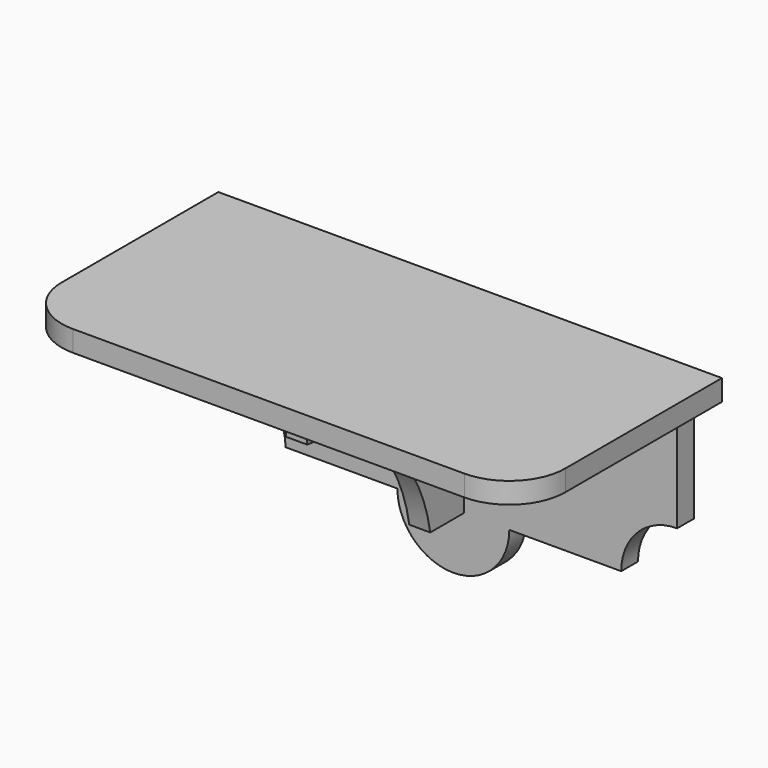
from build123d import *

# Parameters (mm, degrees)
F1_DEPTH = 9.525
F3_DEPTH = 88.9
F5_DEPTH = 9.525
F7_DEPTH = 9.525


# Not quite as in the source:
# - a length typed as a fraction of an inch, garbled in the dataset ("3 / 203.2 mm" for 3/8 in), is restored


with BuildPart() as f1:
    # F0 (on Front) → F1 (new body)
    with BuildSketch(Plane.XZ):
        with BuildLine():
            Line((203.2, 0), (0, 0))
            Line((0, 0), (0, -50.8))
            ThreePointArc((0, -50.8), (17.9605122421, -58.2394877579), (25.4, -76.2))
            Line((25.4, -76.2), (76.2, -76.2))
            ThreePointArc((76.2, -76.2), (101.6, -101.6), (127, -76.2))
            Line((127, -76.2), (177.8, -76.2))
            ThreePointArc((177.8, -76.2), (185.2394877579, -58.2394877579), (203.2, -50.8))
            Line((203.2, -50.8), (203.2, 0))
        make_face()
    extrude(amount=F1_DEPTH)

    # F2 (on face) → F3 (join)
    with BuildSketch(Plane.XZ.offset(9.525)):
        Polygon((96.8375, 0), (96.8375, -76.2), (101.6, -76.2), (106.3625, -76.2), (106.3625, 0), align=None)
    extrude(amount=F3_DEPTH)

    # F4 (on face) → F5 (cut)
    with BuildSketch(Plane.YZ.offset(106.3625)):
        with BuildLine():
            Line((-98.425, -76.2), (-28.575, -76.2))
            ThreePointArc((-28.575, -76.2), (-52.4826849385, -32.3309534324), (-98.425, -12.7))
            Line((-98.425, -12.7), (-98.425, -76.2))
        make_face()
    extrude(amount=-F5_DEPTH, mode=Mode.SUBTRACT)

    # F6 (on face) → F7 (join)
    with BuildSketch(Plane.XY):
        with BuildLine():
            Line((0, -9.525), (0, 0))
            Line((0, 0), (-12.7, 0))
            Line((-12.7, 0), (-12.7, -88.9))
            ThreePointArc((-12.7, -88.9), (-5.2605122421, -106.8605122421), (12.7, -114.3))
            Line((12.7, -114.3), (190.5, -114.3))
            ThreePointArc((190.5, -114.3), (208.4605122421, -106.8605122421), (215.9, -88.9))
            Line((215.9, -88.9), (215.9, 0))
            Line((215.9, 0), (203.2, 0))
            Line((203.2, 0), (203.2, -9.525))
            Line((203.2, -9.525), (106.3625, -9.525))
            Line((106.3625, -9.525), (106.3625, -98.425))
            Line((106.3625, -98.425), (96.8375, -98.425))
            Line((96.8375, -98.425), (96.8375, -9.525))
            Line((96.8375, -9.525), (0, -9.525))
        make_face()
        Polygon((203.2, 0), (0, 0), (0, -9.525), (96.8375, -9.525), (96.8375, -98.425), (106.3625, -98.425), (106.3625, -9.525), (203.2, -9.525), align=None)
    extrude(amount=F7_DEPTH)


solid = f1.part
